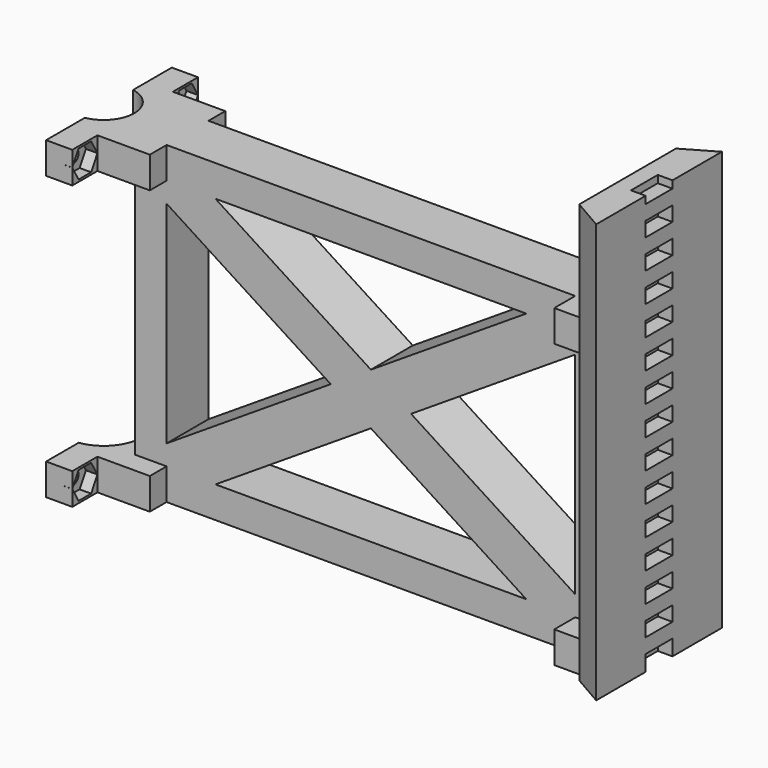
from build123d import *

# Parameters (mm, degrees)
F1_DEPTH  = 6.35
F0_W      = 11.43
F0_H      = 7.62
F0_W_2    = 7.62
F2_DEPTH  = 19.05
F3_DEPTH  = 19.05
F4_DEPTH  = 12.7
F6_DEPTH  = 127
F8_D      = 18.542
F8_DEPTH  = 7.62
F8_TIP    = 5.570578799
F10_D     = 14.8336
F10_DEPTH = 7.62
F10_TIP   = 4.4564630392
F11_W     = 8.128
F11_H     = 1.778
F11_H_2   = 3.556
F11_H_3   = 3.81
F12_DEPTH = 3.556
F9_W      = 12.7
F9_H      = 7.62
F15_DEPTH = 76.201
F13_R     = 1.5875
F14_R     = 1.5875
F16_DEPTH = 38.1
F18_R     = 1.5875
F20_R     = 1.5875
F19_R     = 1.5875
F21_DEPTH = 2.794
F22_DEPTH = 2.794


# Not quite as in the source:
# - a feature names something its author has since deleted; it is built from what else it names


with BuildPart() as f1:
    # F0 (on Front) → F1 (new body, symmetric)
    with BuildSketch(Plane.XZ):
        Polygon((49.53, 38.1), (-49.53, 38.1), (-37.6766666667, 30.48), (37.6766666667, 30.48), align=None)
        Polygon((-37.6766666667, -30.48), (-49.53, -38.1), (49.53, -38.1), (37.6766666667, -30.48), align=None)
        Polygon((-49.53, 25.5814285714), (-57.15, 30.48), (-57.15, -30.48), (-49.53, -25.5814285714), align=None)
        Polygon((-49.53, 30.48), (-57.15, 30.48), (-49.53, 25.5814285714), align=None)
        Polygon((-37.6766666667, 30.48), (-49.53, 38.1), (-49.53, 30.48), align=None)
        Polygon((49.53, 30.48), (49.53, 38.1), (37.6766666667, 30.48), align=None)
        Polygon((37.6766666667, -30.48), (49.53, -38.1), (49.53, -30.48), align=None)
        Polygon((-37.6766666667, -30.48), (-49.53, -30.48), (-49.53, -38.1), align=None)
        Polygon((-49.53, -25.5814285714), (-57.15, -30.48), (-49.53, -30.48), align=None)
        Polygon((57.15, -30.48), (57.15, 30.48), (49.53, 25.5814285714), (49.53, -25.5814285714), align=None)
        Polygon((49.53, -30.48), (57.15, -30.48), (49.53, -25.5814285714), align=None)
        Polygon((57.15, 30.48), (49.53, 30.48), (49.53, 25.5814285714), align=None)
        Polygon((49.53, 25.5814285714), (49.53, 30.48), (37.6766666667, 30.48), (0, 6.2592857143), (9.7366666667, 0), align=None)
        Polygon((49.53, -25.5814285714), (9.7366666667, 0), (0, -6.2592857143), (37.6766666667, -30.48), (49.53, -30.48), align=None)
        Polygon((-49.53, -25.5814285714), (-49.53, -30.48), (-37.6766666667, -30.48), (0, -6.2592857143), (-9.7366666667, 0), align=None)
        Polygon((-37.6766666667, 30.48), (-49.53, 30.48), (-49.53, 25.5814285714), (-9.7366666667, 0), (0, 6.2592857143), align=None)
        Polygon((9.7366666667, 0), (0, 6.2592857143), (-9.7366666667, 0), (0, -6.2592857143), align=None)
    extrude(amount=F1_DEPTH, both=True)

    # F0 (on Front) → F2 (join, symmetric)
    with BuildSketch(Plane.XZ):
        with Locations((-62.865, -34.29)):
            Rectangle(F0_W, F0_H)
        with Locations((-62.865, 34.29)):
            Rectangle(F0_W, F0_H)
        with Locations((-53.34, -34.29)):
            Rectangle(F0_W_2, F0_H)
        with Locations((-53.34, 34.29)):
            Rectangle(F0_W_2, F0_H)
    extrude(amount=F2_DEPTH, both=True)

    # F0 (on Front) → F3 (join, symmetric)
    with BuildSketch(Plane.XZ):
        Polygon((57.15, 63.5), (57.15, 38.1), (57.15, 30.48), (57.15, -30.48), (57.15, -38.1), (64.77, -38.1), (64.77, 63.5), align=None)
    extrude(amount=F3_DEPTH, both=True)

    # F0 (on Front) → F4 (join, symmetric)
    with BuildSketch(Plane.XZ):
        with Locations((53.34, 34.29)):
            Rectangle(F0_W_2, F0_H)
        with Locations((53.34, -34.29)):
            Rectangle(F0_W_2, F0_H)
    extrude(amount=F4_DEPTH, both=True)

    # F5 (on face) → F6 (cut)
    with BuildSketch(Plane.XY.offset(63.5)):
        Polygon((57.15, 14.6505909488), (64.77, 19.05), (57.15, 19.05), align=None)
        Polygon((57.15, -19.05), (64.77, -19.05), (57.15, -14.6505909488), align=None)
    extrude(amount=-F6_DEPTH, mode=Mode.SUBTRACT)

    # F8
    with Locations(Plane(origin=(0, 0, -38.1), x_dir=(1, 0, 0), z_dir=(0, 0, -1))):
        with Locations((-69.85, 0)):
            Hole(F8_D / 2, depth=F8_DEPTH)
            with Locations((0, 0, -(F8_DEPTH + F8_TIP / 2))):  # 118° drill point
                Cone(0, F8_D / 2, F8_TIP, mode=Mode.SUBTRACT)

    # F10
    with Locations(Plane.XY.offset(38.1)):
        with Locations((-69.85, 0)):
            Hole(F10_D / 2, depth=F10_DEPTH)
            with Locations((0, 0, -(F10_DEPTH + F10_TIP / 2))):  # 118° drill point
                Cone(0, F10_D / 2, F10_TIP, mode=Mode.SUBTRACT)

    # F11 (on face) → F12 (cut)
    with BuildSketch(Plane.YZ.offset(64.77)):
        with Locations((0, 62.611)):
            Rectangle(F11_W, F11_H)
        with Locations((0, 56.388)):
            Rectangle(F11_W, F11_H_2)
        with Locations((0, 49.276)):
            Rectangle(F11_W, F11_H_2)
        with Locations((0, 42.164)):
            Rectangle(F11_W, F11_H_2)
        with Locations((0, 35.052)):
            Rectangle(F11_W, F11_H_2)
        with Locations((0, 27.94)):
            Rectangle(F11_W, F11_H_2)
        with Locations((0, 20.828)):
            Rectangle(F11_W, F11_H_2)
        with Locations((0, 13.716)):
            Rectangle(F11_W, F11_H_2)
        with Locations((0, 6.604)):
            Rectangle(F11_W, F11_H_2)
        with Locations((0, -0.508)):
            Rectangle(F11_W, F11_H_2)
        with Locations((0, -7.62)):
            Rectangle(F11_W, F11_H_2)
        with Locations((0, -14.732)):
            Rectangle(F11_W, F11_H_2)
        with Locations((0, -21.844)):
            Rectangle(F11_W, F11_H_2)
        with Locations((0, -28.956)):
            Rectangle(F11_W, F11_H_2)
        with Locations((0, -36.195)):
            Rectangle(F11_W, F11_H_3)
    extrude(amount=-F12_DEPTH, mode=Mode.SUBTRACT)

    # F9 (on face) → F15 (cut, through all)
    with BuildSketch(Plane.XY.offset(38.1)):
        with Locations((-55.88, 15.24)):
            Rectangle(F9_W, F9_H)
        with Locations((-55.88, -15.24)):
            Rectangle(F9_W, F9_H)
    extrude(amount=-F15_DEPTH, mode=Mode.SUBTRACT)

    # F13 (on face) + F14 (on face) → F16 (cut)
    with BuildSketch(Plane(origin=(-68.58, 0, 0), x_dir=(0, -1, 0), z_dir=(-1, 0, 0))):
        with Locations((-15.24, 34.29)):
            Circle(F13_R)
        with Locations((15.24, 34.29)):
            Circle(F13_R)
    with BuildSketch(Plane(origin=(-68.58, 0, 0), x_dir=(0, -1, 0), z_dir=(-1, 0, 0))):
        with Locations((15.24, -34.29)):
            Circle(F14_R)
        with Locations((-15.24, -34.29)):
            Circle(F14_R)
    extrude(amount=-F16_DEPTH, mode=Mode.SUBTRACT)

    # F17 (on face) + F18 (on face) + F20 (on face) + F19 (on face) → F21 (cut)
    with BuildSketch(Plane.YZ.offset(-62.23)):
        Polygon((19.0528211777, 34.29), (17.1464105889, 37.592), (13.3335894111, 37.592), (11.4271788223, 34.29), (13.3335894111, 30.988), (17.1464105889, 30.988), align=None)
    with BuildSketch(Plane.YZ.offset(-62.23)):
        Polygon((-11.43, 34.2948864232), (-13.3335894111, 37.592), (-17.1464105889, 37.592), (-19.05, 34.2948864232), (-19.05, 34.2851135768), (-17.1464105889, 30.988), (-13.3335894111, 30.988), (-11.43, 34.2851135768), align=None)
        with Locations((-15.24, 34.29)):
            Circle(F18_R, mode=Mode.SUBTRACT)
    with BuildSketch(Plane.YZ.offset(-62.23)):
        Polygon((-11.43, -34.2851135768), (-13.3335894111, -30.988), (-17.1464105889, -30.988), (-19.05, -34.2851135768), (-19.05, -34.2948864232), (-17.1464105889, -37.592), (-13.3335894111, -37.592), (-11.43, -34.2948864232), align=None)
        with Locations((-15.24, -34.29)):
            Circle(F20_R, mode=Mode.SUBTRACT)
    with BuildSketch(Plane.YZ.offset(-62.23)):
        Polygon((19.05, -34.2851135768), (17.1464105889, -30.988), (13.3335894111, -30.988), (11.43, -34.2851135768), (11.43, -34.2948864232), (13.3335894111, -37.592), (17.1464105889, -37.592), (19.05, -34.2948864232), align=None)
        with Locations((15.24, -34.29)):
            Circle(F19_R, mode=Mode.SUBTRACT)
    extrude(amount=-F21_DEPTH, mode=Mode.SUBTRACT)

    # F18 (on face) → F22 (cut)
    with BuildSketch(Plane.YZ.offset(-62.23)):
        Polygon((-11.4271788223, 34.29), (-13.3335894111, 37.592), (-17.1464105889, 37.592), (-19.0528211777, 34.29), (-17.1464105889, 30.988), (-13.3335894111, 30.988), align=None)
    extrude(amount=-F22_DEPTH, mode=Mode.SUBTRACT)


solid = f1.part
